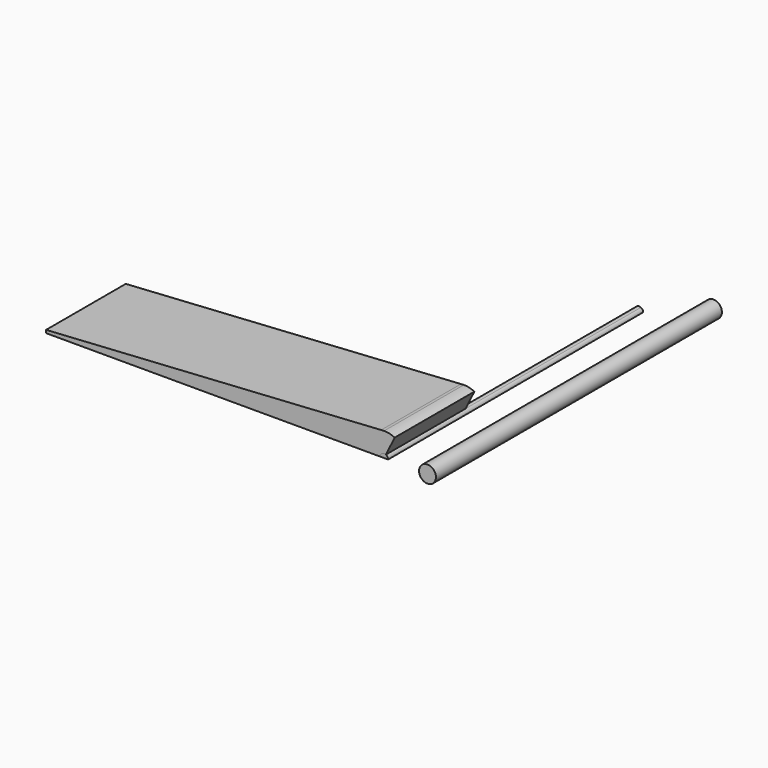
from build123d import *

# Parameters (mm, degrees)
F1_DEPTH = 80
F2_R     = 2.12
F3_DEPTH = 89.7
F4_DEPTH = 25


with BuildPart() as f1:
    # F0 (on Front) → F1 (new body)
    with BuildSketch(Plane.XZ):
        with BuildLine():
            Line((0, 0), (0.4414786382, 0.8972717604))
            ThreePointArc((0.4414786382, 0.8972717604), (-0.5284512096, 0.8489636736), (-1, 0))
            Line((-1, 0), (0, 0))
        make_face()
        with BuildLine():
            ThreePointArc((1, 0), (0.8489636736, 0.5284512096), (0.4414786382, 0.8972717604))
            Line((0.4414786382, 0.8972717604), (0, 0))
            Line((0, 0), (1, 0))
        make_face()
    extrude(amount=-F1_DEPTH)


with BuildPart() as f3:
    # F2 (on Front) → F3 (new body)
    with BuildSketch(Plane.XZ):
        with Locations((10.8834160492, 0)):
            Circle(F2_R)
    extrude(amount=-F3_DEPTH)


with BuildPart() as f4:
    # F0 (on Front) → F4 (new body)
    with BuildSketch(Plane.XZ):
        with BuildLine():
            Line((0.4414786382, 0.8972717604), (2.6488718294, 5.3836305623))
            ThreePointArc((2.6488718294, 5.3836305623), (1.3598192208, 5.8438764264), (0, 6))
            Line((0, 6), (-0.7418538472, 5.9539611075))
            Line((-0.7418538472, 5.9539611075), (-84.8367888957, 0.7350926058))
            Line((-84.8367888957, 0.7350926058), (-84.8367888957, 0))
            Line((-84.8367888957, 0), (-1, 0))
            ThreePointArc((-1, 0), (-0.5284512096, 0.8489636736), (0.4414786382, 0.8972717604))
        make_face()
    extrude(amount=-F4_DEPTH)


solid = Compound([f1.part, f3.part, f4.part])
